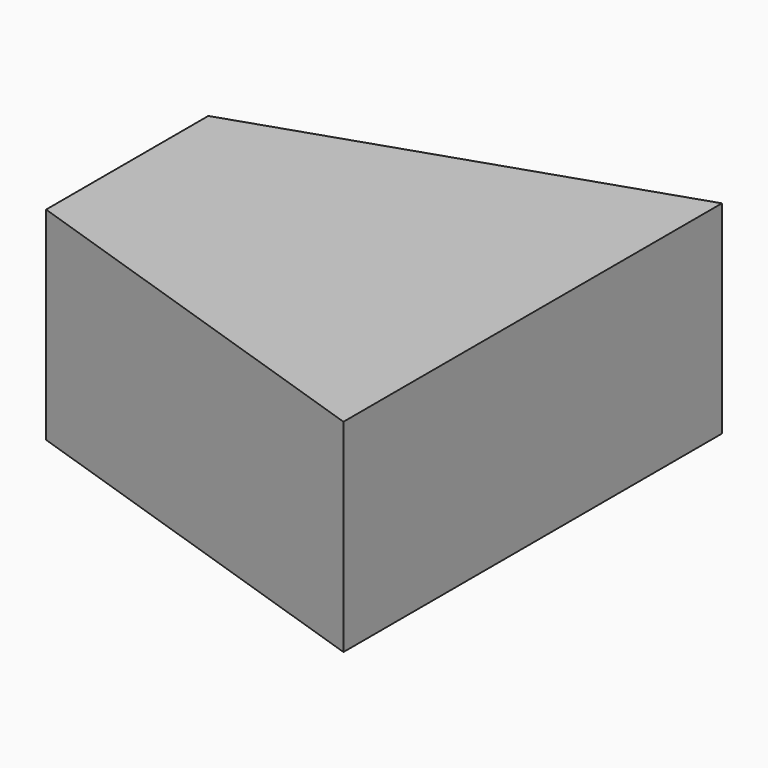
from build123d import *

# Parameters (mm, degrees)
F0_W        = 76.2
F0_H        = 25.4
F1_DEPTH    = 50.8
F2_T1_DEPTH = 420.8872980239


# Not quite as in the source:
# - a fillet or chamfer that OpenCascade refuses, or shapes differently, is made with other operations: its cross-section is extruded or revolved along the edge and cut away or added


with BuildPart() as f1:
    # F0 (on Right) → F1 (new body)
    with BuildSketch(Plane.YZ):
        with Locations((5.0434416714, 12.3206977732)):
            Rectangle(F0_W, F0_H)
    extrude(amount=F1_DEPTH)

    # F2: chamfer of 76.2 x 25.4 on 2 edges, made by hand

    # F2_s2 → F2_t1 (cut)
    with BuildSketch(Plane.XY.offset(-198.1229512387)):
        Polygon((76.2, -33.0565583286), (0, -7.6565583286), (0, -33.0565583286), align=None)
        Polygon((76.2, 43.1434416714), (0, 17.7434416714), (0, 43.1434416714), align=None)
    extrude(amount=F2_T1_DEPTH, mode=Mode.SUBTRACT)


solid = f1.part
